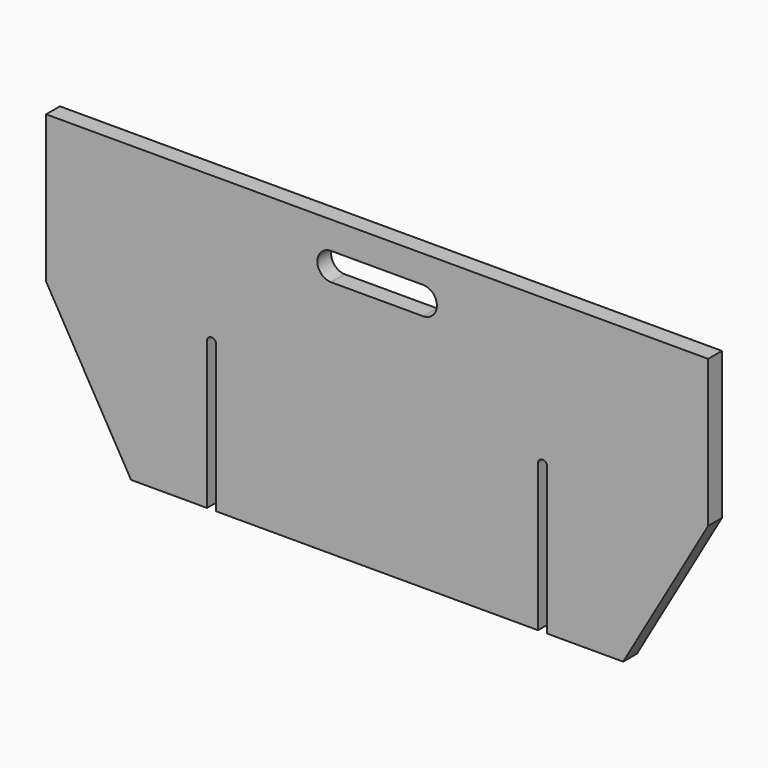
from build123d import *

# Parameters (mm, degrees)
F2_DEPTH = 11.90625
F3_DEPTH = 11.90625


# Not quite as in the source:
# - a variable given as a bare number and used for a length is read in inches; the dataset says mm whatever the document's units were


with BuildPart() as f2:
    # F1 (on Front) → F2 (new body)
    with BuildSketch(Plane.XZ):
        with BuildLine():
            Line((914.4, 406.4), (0, 406.4))
            Line((0, 406.4), (0, 203.2))
            Line((0, 203.2), (117.3175746993, 0))
            Line((117.3175746993, 0), (222.25, 0))
            Line((222.25, 0), (222.25, 203.2))
            ThreePointArc((222.25, 203.2), (228.6, 209.55), (234.95, 203.2))
            Line((234.95, 203.2), (234.95, 0))
            Line((234.95, 0), (679.45, 0))
            Line((679.45, 0), (679.45, 203.2))
            ThreePointArc((679.45, 203.2), (685.8, 209.55), (692.15, 203.2))
            Line((692.15, 203.2), (692.15, 0))
            Line((692.15, 0), (797.0824253007, 0))
            Line((797.0824253007, 0), (914.4, 203.2))
            Line((914.4, 203.2), (914.4, 406.4))
        make_face()
        with BuildLine():
            Line((393.7, 368.3), (457.2, 368.3))
            Line((457.2, 368.3), (520.7, 368.3))
            ThreePointArc((520.7, 368.3), (539.75, 349.25), (520.7, 330.2))
            Line((520.7, 330.2), (457.2, 330.2))
            Line((457.2, 330.2), (393.7, 330.2))
            ThreePointArc((393.7, 330.2), (374.65, 349.25), (393.7, 368.3))
        make_face(mode=Mode.SUBTRACT)
    extrude(amount=F2_DEPTH)

    # F3 (add): a face of the model
    f3_faces = [f2.faces().sort_by_distance(p)[0] for p in [
        (457.2, -11.90625, 211.7591892525),
    ]]
    extrude(f3_faces, amount=F3_DEPTH)


solid = f2.part
